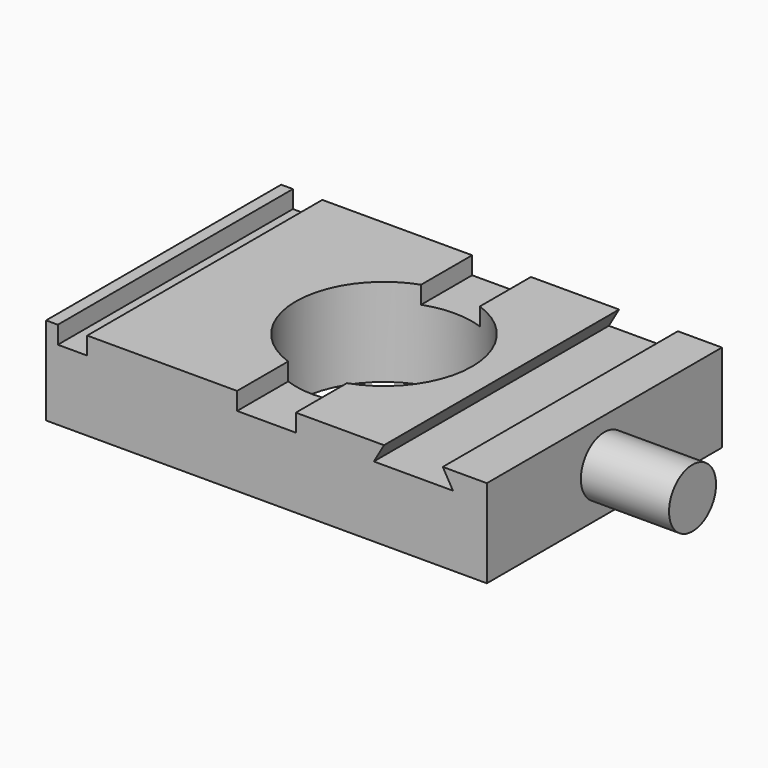
from build123d import *

# Parameters (mm, degrees)
F0_W     = 75
F0_H     = 50
F0_R     = 15
F1_DEPTH = 15
F2_W     = 5
F2_H     = 50
F3_DEPTH = 3
F5_DEPTH = 50.001
F6_R     = 5
F7_DEPTH = 15


with BuildPart() as f1:
    # F0 (on Top) → F1 (new body)
    with BuildSketch(Plane.XY):
        Rectangle(F0_W, F0_H)
        Circle(F0_R, mode=Mode.SUBTRACT)
    extrude(amount=F1_DEPTH)

    # F2 (on face) → F3 (cut)
    with BuildSketch(Plane.XY.offset(15)):
        with Locations((-33, 0)):
            Rectangle(F2_W, F2_H)
        with BuildLine():
            Line((5, 25), (-5, 25))
            Line((-5, 25), (-5, 14.1421356237))
            ThreePointArc((-5, 14.1421356237), (0, 15), (5, 14.1421356237))
            Line((5, 14.1421356237), (5, 25))
        make_face()
        with BuildLine():
            Line((-5, -14.1421356237), (-5, -25))
            Line((-5, -25), (5, -25))
            Line((5, -25), (5, -14.1421356237))
            ThreePointArc((5, -14.1421356237), (0, -15), (-5, -14.1421356237))
        make_face()
    extrude(amount=-F3_DEPTH, mode=Mode.SUBTRACT)

    # F4 (on face) → F5 (cut, through all)
    with BuildSketch(Plane.XZ.offset(25)):
        Polygon((30, 15), (20, 15), (18.2679491924, 12), (31.7320508076, 12), align=None)
    extrude(amount=-F5_DEPTH, mode=Mode.SUBTRACT)

    # F6 (on face) → F7 (join)
    with BuildSketch(Plane.YZ.offset(37.5)):
        with Locations((0, 7.5)):
            Circle(F6_R)
    extrude(amount=F7_DEPTH)


solid = f1.part
